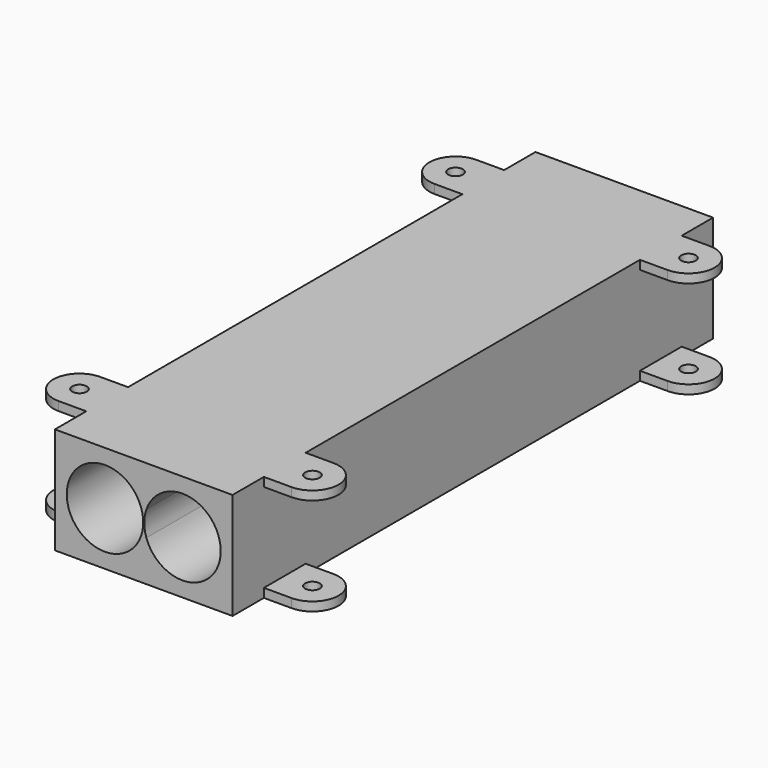
from build123d import *

# Parameters (mm, degrees)
F0_R     = 1.778
F1_DEPTH = 2.159
F2_W     = 43.18
F2_H     = 146.05
F3_DEPTH = 21.59
F4_R     = 1.778
F5_DEPTH = 2.159
F7_DEPTH = 146.051


# Not quite as in the source:
# - a pattern or mirror of a feature is missing from the dataset's text; its kind, count and spacing are read off the source's solid


with BuildPart() as f1:
    # F0 (on Top) → F1 (new body)
    with BuildSketch(Plane.XY):
        Polygon((21.59, 63.5), (21.59, 73.025), (-21.59, 73.025), (-21.59, 63.5), (-21.59, 50.8), (-21.59, -50.8), (-21.59, -63.5), (-21.59, -73.025), (21.59, -73.025), (21.59, -63.5), (21.59, -50.8), (21.59, 50.8), align=None)
        with BuildLine():
            Line((28.321, 63.5), (21.59, 63.5))
            Line((21.59, 63.5), (21.59, 50.8))
            Line((21.59, 50.8), (28.321, 50.8))
            ThreePointArc((28.321, 50.8), (34.671, 57.15), (28.321, 63.5))
        make_face()
        with Locations((28.321, 57.15)):
            Circle(F0_R, mode=Mode.SUBTRACT)
        with BuildLine():
            Line((-21.59, 50.8), (-21.59, 63.5))
            Line((-21.59, 63.5), (-28.321, 63.5))
            ThreePointArc((-28.321, 63.5), (-34.671, 57.15), (-28.321, 50.8))
            Line((-28.321, 50.8), (-21.59, 50.8))
        make_face()
        with Locations((-28.321, 57.15)):
            Circle(F0_R, mode=Mode.SUBTRACT)
        with BuildLine():
            Line((28.321, -50.8), (21.59, -50.8))
            Line((21.59, -50.8), (21.59, -63.5))
            Line((21.59, -63.5), (28.321, -63.5))
            ThreePointArc((28.321, -63.5), (34.671, -57.15), (28.321, -50.8))
        make_face()
        with Locations((28.321, -57.15)):
            Circle(F0_R, mode=Mode.SUBTRACT)
        with BuildLine():
            Line((-21.59, -63.5), (-21.59, -50.8))
            Line((-21.59, -50.8), (-28.321, -50.8))
            ThreePointArc((-28.321, -50.8), (-34.671, -57.15), (-28.321, -63.5))
            Line((-28.321, -63.5), (-21.59, -63.5))
        make_face()
        with Locations((-28.321, -57.15)):
            Circle(F0_R, mode=Mode.SUBTRACT)
    extrude(amount=F1_DEPTH)


with BuildPart() as f1_copies_1:
    # F1_copies: instance of F1
    add(f1.part.mirror(Plane.XY.offset(12.954)))


with BuildPart() as f1_1:
    add(f1.part)

    add(f1_copies_1.part)  # F3 merges F1_copies_1
    # F2 (on face) → F3 (join)
    with BuildSketch(Plane.XY.offset(2.159)):
        Rectangle(F2_W, F2_H)
    extrude(amount=F3_DEPTH)

    # F4 (on face) → F5 (join)
    with BuildSketch(Plane.XY):
        Polygon((21.59, 63.5), (21.59, 73.025), (-21.59, 73.025), (-21.59, 63.5), (-21.59, 50.8), (-21.59, -50.8), (-21.59, -63.5), (-21.59, -73.025), (21.59, -73.025), (21.59, -63.5), (21.59, -50.8), (21.59, 50.8), align=None)
        with BuildLine():
            Line((28.321, 63.5), (21.59, 63.5))
            Line((21.59, 63.5), (21.59, 50.8))
            Line((21.59, 50.8), (28.321, 50.8))
            ThreePointArc((28.321, 50.8), (34.671, 57.15), (28.321, 63.5))
        make_face()
        with Locations((28.321, 57.15)):
            Circle(F4_R, mode=Mode.SUBTRACT)
        with BuildLine():
            Line((-21.59, 50.8), (-21.59, 63.5))
            Line((-21.59, 63.5), (-28.321, 63.5))
            ThreePointArc((-28.321, 63.5), (-34.671, 57.15), (-28.321, 50.8))
            Line((-28.321, 50.8), (-21.59, 50.8))
        make_face()
        with Locations((-28.321, 57.15)):
            Circle(F4_R, mode=Mode.SUBTRACT)
        with BuildLine():
            Line((28.321, -50.8), (21.59, -50.8))
            Line((21.59, -50.8), (21.59, -63.5))
            Line((21.59, -63.5), (28.321, -63.5))
            ThreePointArc((28.321, -63.5), (34.671, -57.15), (28.321, -50.8))
        make_face()
        with Locations((28.321, -57.15)):
            Circle(F4_R, mode=Mode.SUBTRACT)
        with BuildLine():
            Line((-21.59, -63.5), (-21.59, -50.8))
            Line((-21.59, -50.8), (-28.321, -50.8))
            ThreePointArc((-28.321, -50.8), (-34.671, -57.15), (-28.321, -63.5))
            Line((-28.321, -63.5), (-21.59, -63.5))
        make_face()
        with Locations((-28.321, -57.15)):
            Circle(F4_R, mode=Mode.SUBTRACT)
    extrude(amount=F5_DEPTH)

    # F6 (on face) → F7 (cut, through all)
    with BuildSketch(Plane.XZ.offset(73.025)):
        with BuildLine():
            Line((-0.635, 9.9229806335), (-0.635, 15.9850193665))
            ThreePointArc((-0.635, 15.9850193665), (-18.7198, 12.954), (-0.635, 9.9229806335))
        make_face()
        with BuildLine():
            ThreePointArc((-0.635, 9.9229806335), (-0.2548795436, 11.4173524802), (-0.127, 12.954))
            ThreePointArc((-0.127, 12.954), (-0.2548795436, 14.4906475198), (-0.635, 15.9850193665))
            Line((-0.635, 15.9850193665), (-0.635, 9.9229806335))
        make_face()
        with BuildLine():
            Line((0.635, 9.9229806335), (0.635, 15.9850193665))
            ThreePointArc((0.635, 15.9850193665), (0.127, 12.954), (0.635, 9.9229806335))
        make_face()
        with BuildLine():
            ThreePointArc((18.7198, 12.954), (10.9600475198, 22.1225204564), (0.635, 15.9850193665))
            Line((0.635, 15.9850193665), (0.635, 9.9229806335))
            ThreePointArc((0.635, 9.9229806335), (10.9600475198, 3.7854795436), (18.7198, 12.954))
        make_face()
    extrude(amount=-F7_DEPTH, mode=Mode.SUBTRACT)


solid = f1_1.part
